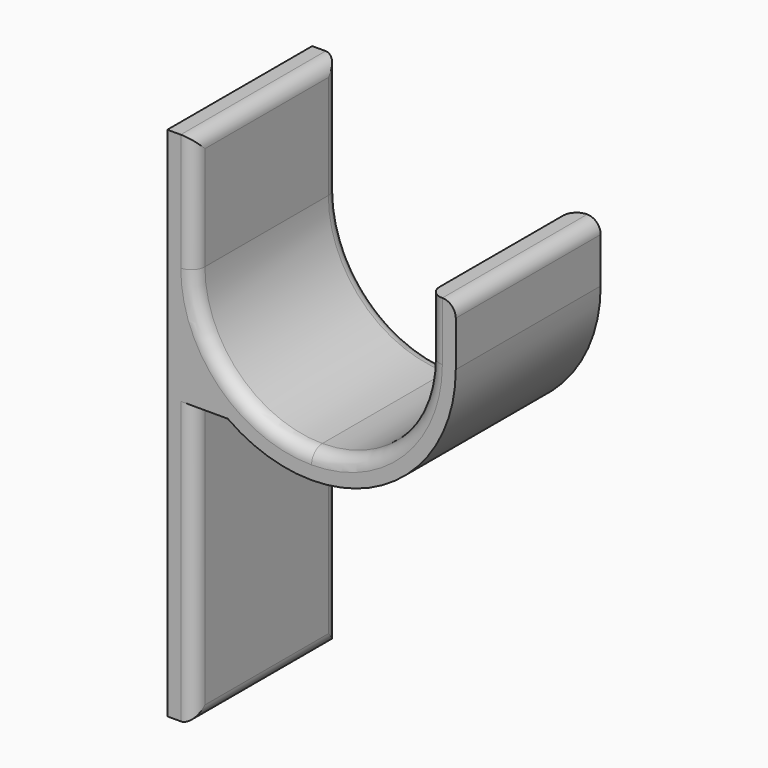
from build123d import *

# Parameters (mm, degrees)
F1_W     = 4
F1_H     = 42
F1_H_2   = 8.75
F2_DEPTH = 27
F3_R     = 1.99999


# Not quite as in the source:
# - a fillet or chamfer is up to 0.001 mm smaller than in the source, because OpenCascade refuses the exact size


with BuildPart() as f2:
    # F1 (on Front) → F2 (new body)
    with BuildSketch(Plane.XZ):
        with BuildLine():
            Line((4, 35), (0, 35))
            Line((0, 35), (0, 17.5))
            ThreePointArc((0, 17.5), (1.0244047706, 24.0574385243), (4, 29.9899959968))
            Line((4, 29.9899959968), (4, 35))
        make_face()
        with BuildLine():
            ThreePointArc((4, 5.0100040032), (1.0244047706, 10.9425614757), (0, 17.5))
            Line((0, 17.5), (0, 0))
            Line((0, 0), (4, 0))
            Line((4, 0), (4, 5.0100040032))
        make_face()
        with BuildLine():
            Line((4, 17.5), (0, 17.5))
            ThreePointArc((0, 17.5), (1.0244047706, 10.9425614757), (4, 5.0100040032))
            Line((4, 5.0100040032), (4, 17.5))
        make_face()
        with BuildLine():
            ThreePointArc((4, 29.9899959968), (1.0244047706, 24.0574385243), (0, 17.5))
            Line((0, 17.5), (4, 17.5))
            Line((4, 17.5), (4, 29.9899959968))
        make_face()
        with Locations((2, -21)):
            Rectangle(F1_W, F1_H)
        with BuildLine():
            ThreePointArc((9.0100040032, 0), (6.2972042045, 2.2972042045), (4, 5.0100040032))
            Line((4, 5.0100040032), (4, 0))
            Line((4, 0), (9.0100040032, 0))
        make_face()
        with BuildLine():
            Line((4, 17.5), (4, 5.0100040032))
            ThreePointArc((4, 5.0100040032), (6.2972042045, 2.2972042045), (9.0100040032, 0))
            Line((9.0100040032, 0), (21.5, 0))
            ThreePointArc((21.5, 0), (9.1256313292, 5.1256313292), (4, 17.5))
        make_face()
        with BuildLine():
            Line((21.5, 0), (9.0100040032, 0))
            ThreePointArc((9.0100040032, 0), (21.5, -4), (33.9899959968, 0))
            Line((33.9899959968, 0), (21.5, 0))
        make_face()
        with BuildLine():
            ThreePointArc((39, 17.5), (33.8743686708, 5.1256313292), (21.5, 0))
            Line((21.5, 0), (33.9899959968, 0))
            ThreePointArc((33.9899959968, 0), (40.6152414833, 7.6583770122), (43, 17.5))
            Line((43, 17.5), (39, 17.5))
        make_face()
        with Locations((41, 21.875)):
            Rectangle(F1_W, F1_H_2)
    extrude(amount=F2_DEPTH)

    # F3 (radius 2 in the source; OpenCascade refuses exactly that, so slightly less here)
    f3_edges = [f2.edges().sort_by_distance(p)[0] for p in [
        (4, -27, -21),
        (4, -27, 26.25),
        (4, 0, -21),
        (4, -13.5, -42),
        (4, 0, 26.25),
        (43, -13.5, 26.25),
        (4, -13.5, 35),
    ]]
    fillet(f3_edges, radius=F3_R)


solid = f2.part
